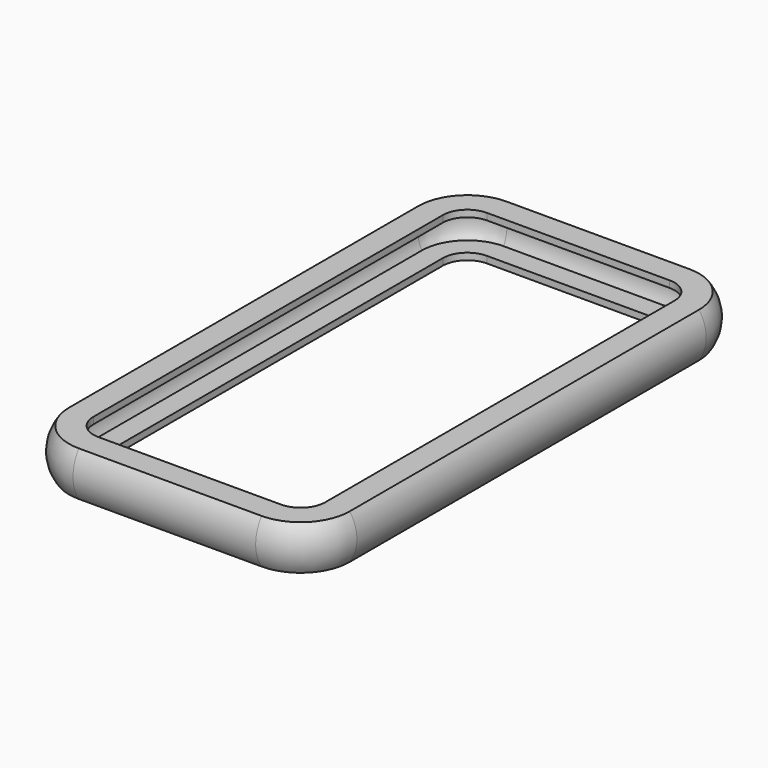
from build123d import *

# Parameters (mm, degrees)
F1_DEPTH  = 5
F3_DEPTH  = 49
F5_DEPTH  = 20.5
F15_DEPTH = 1.5
F17_T     = 1.5


# Not quite as in the source:
# - a shell that OpenCascade refuses in one call is made with other operations: the cavity is built on its own and cut out


with BuildPart() as f1:
    # F0 (on Top) → F1 (new body, symmetric)
    with BuildSketch(Plane.XY):
        with BuildLine():
            Line((31.5, -49), (31.5, 49))
            ThreePointArc((31.5, 49), (28.2781745931, 56.7781745931), (20.5, 60))
            Line((20.5, 60), (-20.5, 60))
            ThreePointArc((-20.5, 60), (-28.2781745931, 56.7781745931), (-31.5, 49))
            Line((-31.5, 49), (-31.5, -49))
            ThreePointArc((-31.5, -49), (-28.2781745931, -56.7781745931), (-20.5, -60))
            Line((-20.5, -60), (20.5, -60))
            ThreePointArc((20.5, -60), (28.2781745931, -56.7781745931), (31.5, -49))
        make_face()
        with BuildLine():
            ThreePointArc((-29.5, 49), (-26.8639610307, 55.3639610307), (-20.5, 58))
            Line((-20.5, 58), (20.5, 58))
            ThreePointArc((20.5, 58), (26.8639610307, 55.3639610307), (29.5, 49))
            Line((29.5, 49), (29.5, -49))
            ThreePointArc((29.5, -49), (26.8639610307, -55.3639610307), (20.5, -58))
            Line((20.5, -58), (-20.5, -58))
            ThreePointArc((-20.5, -58), (-26.8639610307, -55.3639610307), (-29.5, -49))
            Line((-29.5, -49), (-29.5, 49))
        make_face(mode=Mode.SUBTRACT)
    extrude(amount=F1_DEPTH, both=True)

    # F2 (on Front) → F3 (join, symmetric)
    with BuildSketch(Plane.XZ):
        with BuildLine():
            Line((-31.5, -5), (-31.5, 5))
            ThreePointArc((-31.5, 5), (-33.1261364576, 0), (-31.5, -5))
        make_face()
        with BuildLine():
            ThreePointArc((31.5, -5), (33.1261364576, 0), (31.5, 5))
            Line((31.5, 5), (31.5, -5))
        make_face()
    extrude(amount=F3_DEPTH, both=True)

    # F4 (on Right) → F5 (join, symmetric)
    with BuildSketch(Plane.YZ):
        with BuildLine():
            ThreePointArc((60, -5), (61.6261364576, 0), (60, 5))
            Line((60, 5), (60, -5))
        make_face()
        with BuildLine():
            Line((-60, -5), (-60, 5))
            ThreePointArc((-60, 5), (-61.6261364576, 0), (-60, -5))
        make_face()
    extrude(amount=F5_DEPTH, both=True)

    # F7: sweep along a path in F0
    with BuildLine(Plane.XY) as f7_path:
        ThreePointArc((-20.5, 62), (-29.6923881554, 58.1923881554), (-33.5, 49))
    # F6 (on face) → F7 (sweep)
    with BuildSketch(Plane(origin=(-20.5, 0, 0), x_dir=(0, -1, 0), z_dir=(-1, 0, 0))):
        with BuildLine():
            ThreePointArc((-60, 5), (-61.6261364576, 0), (-60, -5))
            Line((-60, -5), (-60, 5))
        make_face()
    sweep(path=f7_path.line)

    # F9: sweep along a path in F0
    with BuildLine(Plane.XY) as f9_path:
        ThreePointArc((33.5, 49), (29.6923881554, 58.1923881554), (20.5, 62))
    # F8 (on face) → F9 (sweep)
    with BuildSketch(Plane.YZ.offset(20.5)):
        with BuildLine():
            Line((60, 5), (60, -5))
            ThreePointArc((60, -5), (61.6261364576, 0), (60, 5))
        make_face()
    sweep(path=f9_path.line)

    # F11: sweep along a path in F0
    with BuildLine(Plane.XY) as f11_path:
        ThreePointArc((20.5, -62), (29.6923881554, -58.1923881554), (33.5, -49))
    # F10 (on face) → F11 (sweep)
    with BuildSketch(Plane.YZ.offset(20.5)):
        with BuildLine():
            Line((-60, -5), (-60, 5))
            ThreePointArc((-60, 5), (-61.6261364576, 0), (-60, -5))
        make_face()
    sweep(path=f11_path.line)

    # F13: sweep along a path in F0
    with BuildLine(Plane.XY) as f13_path:
        ThreePointArc((-33.5, -49), (-29.6923881554, -58.1923881554), (-20.5, -62))
    # F12 (on face) → F13 (sweep)
    with BuildSketch(Plane(origin=(-20.5, 0, 0), x_dir=(0, -1, 0), z_dir=(-1, 0, 0))):
        with BuildLine():
            ThreePointArc((60, -5), (61.6261364576, 0), (60, 5))
            Line((60, 5), (60, -5))
        make_face()
    sweep(path=f13_path.line)

    # F14 (on face) → F15 (join)
    with BuildSketch(Plane.XY.offset(5)):
        with BuildLine():
            Line((20.5, 60), (-20.5, 60))
            ThreePointArc((-20.5, 60), (-28.2781745931, 56.7781745931), (-31.5, 49))
            Line((-31.5, 49), (-31.5, -49))
            ThreePointArc((-31.5, -49), (-28.2781745931, -56.7781745931), (-20.5, -60))
            Line((-20.5, -60), (20.5, -60))
            ThreePointArc((20.5, -60), (28.2781745931, -56.7781745931), (31.5, -49))
            Line((31.5, -49), (31.5, 49))
            ThreePointArc((31.5, 49), (28.2781745931, 56.7781745931), (20.5, 60))
        make_face()
        with BuildLine():
            Line((-29.5, -49), (-29.5, 49))
            ThreePointArc((-29.5, 49), (-26.8639610307, 55.3639610307), (-20.5, 58))
            Line((-20.5, 58), (20.5, 58))
            ThreePointArc((20.5, 58), (26.8639610307, 55.3639610307), (29.5, 49))
            Line((29.5, 49), (29.5, -49))
            ThreePointArc((29.5, -49), (26.8639610307, -55.3639610307), (20.5, -58))
            Line((20.5, -58), (-20.5, -58))
            ThreePointArc((-20.5, -58), (-26.8639610307, -55.3639610307), (-29.5, -49))
        make_face(mode=Mode.SUBTRACT)
        with BuildLine():
            ThreePointArc((-20.5, 58), (-26.8639610307, 55.3639610307), (-29.5, 49))
            Line((-29.5, 49), (-29.5, -49))
            ThreePointArc((-29.5, -49), (-26.8639610307, -55.3639610307), (-20.5, -58))
            Line((-20.5, -58), (20.5, -58))
            ThreePointArc((20.5, -58), (26.8639610307, -55.3639610307), (29.5, -49))
            Line((29.5, -49), (29.5, 49))
            ThreePointArc((29.5, 49), (26.8639610307, 55.3639610307), (20.5, 58))
            Line((20.5, 58), (-20.5, 58))
        make_face()
        with BuildLine():
            ThreePointArc((-26, 49), (-24.3890872965, 52.8890872965), (-20.5, 54.5))
            Line((-20.5, 54.5), (20.5, 54.5))
            ThreePointArc((20.5, 54.5), (24.3890872965, 52.8890872965), (26, 49))
            Line((26, 49), (26, -49))
            ThreePointArc((26, -49), (24.3890872965, -52.8890872965), (20.5, -54.5))
            Line((20.5, -54.5), (-20.5, -54.5))
            ThreePointArc((-20.5, -54.5), (-24.3890872965, -52.8890872965), (-26, -49))
            Line((-26, -49), (-26, 49))
        make_face(mode=Mode.SUBTRACT)
    extrude(amount=-F15_DEPTH)

    # F16: F1 across plane


with BuildPart() as f1_1:
    add(f1.part)
    add(f1.part.mirror(Plane.XY))

    # F17: shell of thickness 1.5, made by hand


with BuildPart() as f17_core1:
    # F17_t2: copy of F1
    add(f1_1.part)

    # the walls: a layer under each face that stays
    f17_faces = [f17_core1.faces().sort_by_distance(p)[0] for p in [
        (-27, -51.4285714286, -5),
        (33.1261364576, 0, 0),
        (29.4280267093, 57.9280267093, 0),
        (0, 61.6261364576, 0),
        (-29.4280267093, 57.9280267093, 0),
        (-33.1261364576, 0, 0),
        (-29.4280267093, -57.9280267093, 0),
        (0, -61.6261364576, 0),
        (29.4280267093, -57.9280267093, 0),
        (-27, -51.4285714286, 5),
        (24.3890872965, -52.8890872965, -4.25),
        (26, 0, -4.25),
        (0, -54.5, -4.25),
        (24.3890872965, 52.8890872965, -4.25),
        (-24.3890872965, -52.8890872965, -4.25),
        (0, 54.5, -4.25),
        (-26, 0, -4.25),
        (-24.3890872965, 52.8890872965, -4.25),
        (-27.5333333333, -54.1333333333, -3.5),
        (24.3890872965, -52.8890872965, 4.25),
        (26, 0, 4.25),
        (0, -54.5, 4.25),
        (24.3890872965, 52.8890872965, 4.25),
        (-24.3890872965, -52.8890872965, 4.25),
        (0, 54.5, 4.25),
        (-26, 0, 4.25),
        (-24.3890872965, 52.8890872965, 4.25),
        (-27.5333333333, -54.1333333333, 3.5),
    ]]
    thicken(f17_faces, amount=-F17_T, mode=Mode.SUBTRACT)


with BuildPart() as f1_2:
    add(f1_1.part)

    # what is left inside the walls is the cavity
    f17_cavity = [f17_core1.part.solids().sort_by_distance(p)[0] for p in [
        (-31.611136, 16.333334, 0),
    ]]
    add(f17_cavity, mode=Mode.SUBTRACT)


solid = f1_2.part
